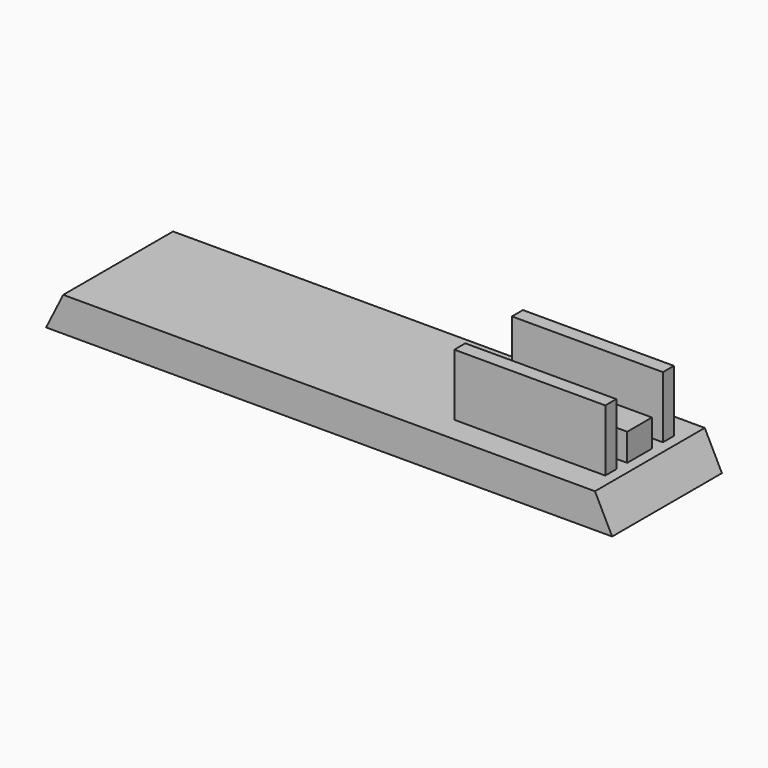
from build123d import *

# Parameters (mm, degrees)
F0_W     = 165
F0_H     = 40
F1_DEPTH = 10
F2_SIZE2 = 9.99999
F2_SIZE  = 4.99999
F3_SIZE2 = 4.99999
F3_SIZE  = 9.99999
F4_W     = 44
F4_H     = 4
F5_DEPTH = 18
F4_H_2   = 9
F6_DEPTH = 8


# Not quite as in the source:
# - a fillet or chamfer is up to 0.001 mm smaller than in the source, because OpenCascade refuses the exact size


with BuildPart() as f1:
    # F0 (on Top) → F1 (new body)
    with BuildSketch(Plane.XY):
        with Locations((82.5, 20)):
            Rectangle(F0_W, F0_H)
    extrude(amount=F1_DEPTH)

    # F2 (size 5 and 10 in the source; OpenCascade refuses exactly that, so slightly less here)
    f2_edges = [f1.edges().sort_by_distance(p)[0] for p in [
        (165, 20, 10),
    ]]
    f2_side = f1.faces().sort_by_distance((82.5, 20, 10))[0]
    chamfer(f2_edges, length=F2_SIZE, length2=F2_SIZE2, reference=f2_side)

    # F3 (size 10 and 5 in the source; OpenCascade refuses exactly that, so slightly less here)
    f3_edges = [f1.edges().sort_by_distance(p)[0] for p in [
        (0, 20, 10),
    ]]
    f3_side = f1.faces().sort_by_distance((0, 20, 5))[0]
    chamfer(f3_edges, length=F3_SIZE, length2=F3_SIZE2, reference=f3_side)

    # F4 (on face) → F5 (join)
    with BuildSketch(Plane.XY.offset(10)):
        with Locations((135, 30.5)):
            Rectangle(F4_W, F4_H)
        with Locations((135, 9.5)):
            Rectangle(F4_W, F4_H)
    extrude(amount=F5_DEPTH)

    # F4 (on face) → F6 (join)
    with BuildSketch(Plane.XY.offset(10)):
        with Locations((135, 20)):
            Rectangle(F4_W, F4_H_2)
    extrude(amount=F6_DEPTH)


solid = f1.part
